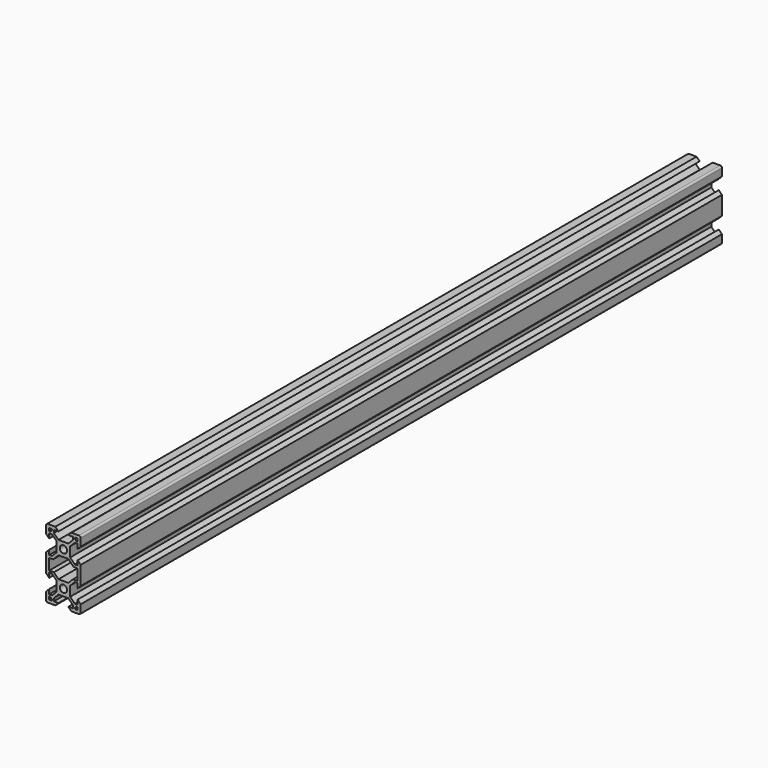
from build123d import *

# Parameters (mm, degrees)
F0_W             = 20
F0_H             = 20
F1_DEPTH         = 463
F2_R             = 2.1
F3_DEPTH         = 463.001
F4_R             = 1
F6_DEPTH         = 463.001
F6_COPIES3_COUNT = 2
F6_COPIES3_ANGLE = 90
F6_COPIES4_COUNT = 2
F6_COPIES4_ANGLE = 270
F6_COPIES6_COUNT = 2
F9_W             = 16.4
F9_H             = 6.8613203436
F10_DEPTH        = 463.001
F12_DEPTH        = 463


# Not quite as in the source:
# - a pattern or mirror of a feature is missing from the dataset's text; its kind, count and spacing are read off the source's solid


with BuildPart() as f1:
    # F0 (on Front) → F1 (new body)
    with BuildSketch(Plane.XZ):
        Rectangle(F0_W, F0_H)
    extrude(amount=F1_DEPTH)

    # F2 (on face) → F3 (cut, through all)
    with BuildSketch(Plane.XZ.offset(463)):
        Circle(F2_R)
    extrude(amount=-F3_DEPTH, mode=Mode.SUBTRACT)

    # F4
    f4_edges = [f1.edges().sort_by_distance(p)[0] for p in [
        (-10, -231.5, 10),
        (10, -231.5, 10),
    ]]
    fillet(f4_edges, radius=F4_R)

    # F5 (on face) → F6 (cut, through all)
    with BuildSketch(Plane.XZ.offset(463)):
        Polygon((0, 3.9006601718), (0, 10), (-2.84, 10), (-4.64, 10), (-2.84, 8.2), (-5.4993398282, 8.2), (-5.4993398282, 6.56), (-2.84, 3.9006601718), align=None)
        Polygon((-6.5693398282, 8.2), (-8.2, 8.2), (-7.0953059148, 7.0953059148), (-6.5693398282, 7.6212720014), align=None)
    f6 = extrude(amount=-F6_DEPTH, mode=Mode.SUBTRACT)

    # F6_copies: F6 across plane
    add(f6.mirror(Plane(origin=(0, 0, 0), x_dir=(-0.7071067812, 0, -0.7071067812), z_dir=(0.7071067812, 0, -0.7071067812))), mode=Mode.SUBTRACT)

    # F6_copies1: F6 across plane
    add(f6.mirror(Plane(origin=(0, 0, 0), x_dir=(0.7071067812, 0, -0.7071067812), z_dir=(-0.7071067812, 0, -0.7071067812))), mode=Mode.SUBTRACT)

    # F6_copies2: F6 across plane
    add(f6.mirror(Plane(origin=(0, 0, 0), x_dir=(0, 0, 1), z_dir=(1, 0, 0))), mode=Mode.SUBTRACT)

    # F6_copies3: F6 ×2 about axis
    f6_copies3_axis = Axis((0, 0, 0), (0, 1, 0))
    for i in range(1, F6_COPIES3_COUNT):
        add(f6.rotate(f6_copies3_axis, i * F6_COPIES3_ANGLE / (F6_COPIES3_COUNT - 1)), mode=Mode.SUBTRACT)

    # F6_copies4: F6 ×2 about axis
    f6_copies4_axis = Axis((0, 0, 0), (0, 1, 0))
    for i in range(1, F6_COPIES4_COUNT):
        add(f6.rotate(f6_copies4_axis, i * F6_COPIES4_ANGLE / (F6_COPIES4_COUNT - 1)), mode=Mode.SUBTRACT)

    # F6_copies5: F6 across plane
    add(f6.mirror(Plane(origin=(0, 0, 0), x_dir=(-1, 0, 0), z_dir=(0, 0, -1))), mode=Mode.SUBTRACT)

    # F6_copies6: F6 ×2 about axis
    f6_copies6_axis = Axis((0, 0, 0), (0, 1, 0))
    for i in range(1, F6_COPIES6_COUNT):
        add(f6.rotate(f6_copies6_axis, i * 360 / F6_COPIES6_COUNT), mode=Mode.SUBTRACT)

    # F8: F1 across face


with BuildPart() as f1_1:
    add(f1.part)
    add(f1.part.mirror(Plane(origin=(-7.32, -231.5, -10), x_dir=(1, 0, 0), z_dir=(0, 0, -1))))

    # F9 (on face) → F10 (cut, through all)
    with BuildSketch(Plane.XZ.offset(463)):
        with Locations((0, -10)):
            Rectangle(F9_W, F9_H)
    extrude(amount=-F10_DEPTH, mode=Mode.SUBTRACT)

    # F11 (on face) → F12 (join, through all)
    with BuildSketch(Plane.XZ.offset(463)):
        with BuildLine():
            ThreePointArc((-9, -10), (-9.7071067812, -9.7071067812), (-10, -9))
            Line((-10, -9), (-10, -11))
            ThreePointArc((-10, -11), (-9.7071067812, -10.2928932188), (-9, -10))
        make_face()
        with BuildLine():
            ThreePointArc((10, -9), (9.7071067812, -9.7071067812), (9, -10))
            ThreePointArc((9, -10), (9.7071067812, -10.2928932188), (10, -11))
            Line((10, -11), (10, -9))
        make_face()
        Polygon((5.9386796564, -6.9993398282), (8.2, -6.9993398282), (8.2, -6.5693398282), (5.5086796564, -6.5693398282), align=None)
        Polygon((-8.2, -6.5693398282), (-8.2, -6.9993398282), (-5.9386796564, -6.9993398282), (-5.5086796564, -6.5693398282), align=None)
    extrude(amount=-F12_DEPTH)


solid = f1_1.part
